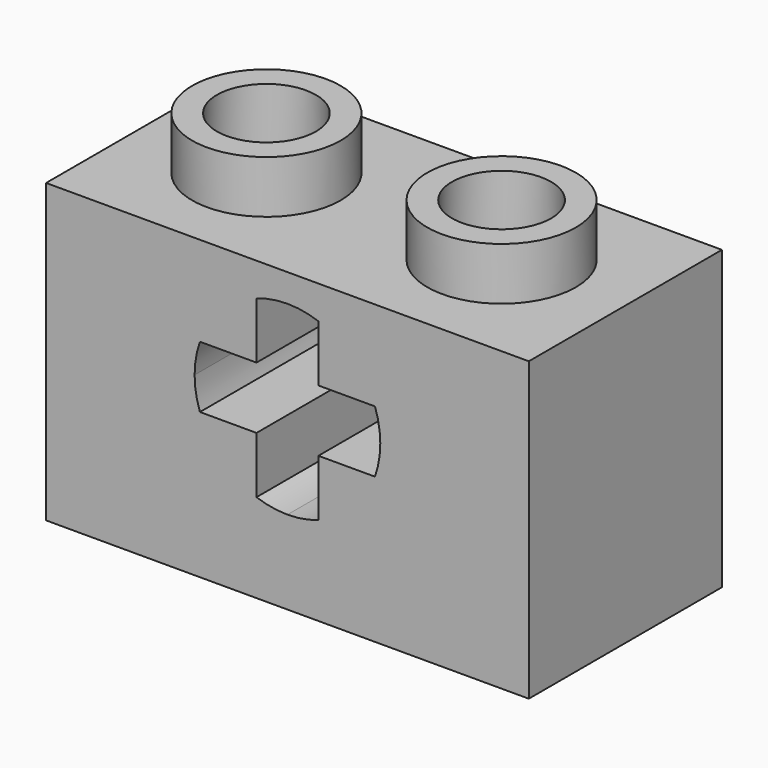
from build123d import *

# Parameters (mm, degrees)
F0_W     = 15.6
F0_H     = 9.6
F1_DEPTH = 7.8
F2_R     = 2.4
F2_R_2   = 1.6
F3_DEPTH = 1.7
F5_DEPTH = 2


# Not quite as in the source:
# - a feature names something its author has since deleted; it is built from what else it names


with BuildPart() as f1:
    # F0 (on Front) → F1 (new body)
    with BuildSketch(Plane.XZ):
        with Locations((7.5497636572, 4.7150965011)):
            Rectangle(F0_W, F0_H)
        with BuildLine():
            Line((10.5497636572, 6.6150965011), (10.5497636572, 5.6150965011))
            Line((10.5497636572, 5.6150965011), (10.5497636572, 4.6150965011))
            Line((10.5497636572, 4.6150965011), (10.3781907819, 4.6150965011))
            ThreePointArc((10.3781907819, 4.6150965011), (9.6710840007, 3.4937761575), (8.5497636572, 2.7866693764))
            Line((8.5497636572, 2.7866693764), (8.5497636572, 2.6150965011))
            Line((8.5497636572, 2.6150965011), (7.5497636572, 2.6150965011))
            Line((7.5497636572, 2.6150965011), (6.5497636572, 2.6150965011))
            Line((6.5497636572, 2.6150965011), (6.5497636572, 2.7866693764))
            ThreePointArc((6.5497636572, 2.7866693764), (5.4284433136, 3.4937761575), (4.7213365324, 4.6150965011))
            Line((4.7213365324, 4.6150965011), (4.5497636572, 4.6150965011))
            Line((4.5497636572, 4.6150965011), (4.5497636572, 5.6150965067))
            Line((4.5497636572, 5.6150965067), (4.5497636572, 6.6150965011))
            Line((4.5497636572, 6.6150965011), (4.7213365324, 6.6150965011))
            ThreePointArc((4.7213365324, 6.6150965011), (5.4284433136, 7.7364168447), (6.5497636572, 8.4435236258))
            Line((6.5497636572, 8.4435236258), (6.5497636572, 8.6150965011))
            Line((6.5497636572, 8.6150965011), (7.5497636572, 8.6150965011))
            Line((7.5497636572, 8.6150965011), (8.5497636572, 8.6150965011))
            Line((8.5497636572, 8.6150965011), (8.5497636572, 8.4435236258))
            ThreePointArc((8.5497636572, 8.4435236258), (9.6710840007, 7.7364168447), (10.3781907819, 6.6150965011))
            Line((10.3781907819, 6.6150965011), (10.5497636572, 6.6150965011))
        make_face(mode=Mode.SUBTRACT)
        with BuildLine():
            ThreePointArc((8.5497636572, 2.7866693764), (9.6710840007, 3.4937761575), (10.3781907819, 4.6150965011))
            Line((10.3781907819, 4.6150965011), (8.5497636572, 4.6150965011))
            Line((8.5497636572, 4.6150965011), (8.5497636572, 2.7866693764))
        make_face()
        with BuildLine():
            Line((8.5497636572, 6.6150965011), (10.3781907819, 6.6150965011))
            ThreePointArc((10.3781907819, 6.6150965011), (9.6710840007, 7.7364168447), (8.5497636572, 8.4435236258))
            Line((8.5497636572, 8.4435236258), (8.5497636572, 6.6150965011))
        make_face()
        with BuildLine():
            Line((4.7213365324, 6.6150965011), (6.5497636572, 6.6150965011))
            Line((6.5497636572, 6.6150965011), (6.5497636572, 8.4435236258))
            ThreePointArc((6.5497636572, 8.4435236258), (5.4284433136, 7.7364168447), (4.7213365324, 6.6150965011))
        make_face()
        with BuildLine():
            Line((6.5497636572, 2.7866693764), (6.5497636572, 4.6150965011))
            Line((6.5497636572, 4.6150965011), (4.7213365324, 4.6150965011))
            ThreePointArc((4.7213365324, 4.6150965011), (5.4284433136, 3.4937761575), (6.5497636572, 2.7866693764))
        make_face()
        with BuildLine():
            Line((10.5497636572, 4.6150965011), (10.5497636572, 5.6150965011))
            ThreePointArc((10.5497636572, 5.6150965011), (10.5065593361, 5.1077905649), (10.3781907819, 4.6150965011))
            Line((10.3781907819, 4.6150965011), (10.5497636572, 4.6150965011))
        make_face()
        with BuildLine():
            ThreePointArc((10.3781907819, 6.6150965011), (10.5065593361, 6.1224024373), (10.5497636572, 5.6150965011))
            Line((10.5497636572, 5.6150965011), (10.5497636572, 6.6150965011))
            Line((10.5497636572, 6.6150965011), (10.3781907819, 6.6150965011))
        make_face()
        with BuildLine():
            ThreePointArc((7.5497636572, 8.6150965011), (8.0570695933, 8.5718921801), (8.5497636572, 8.4435236258))
            Line((8.5497636572, 8.4435236258), (8.5497636572, 8.6150965011))
            Line((8.5497636572, 8.6150965011), (7.5497636572, 8.6150965011))
        make_face()
        with BuildLine():
            ThreePointArc((6.5497636572, 8.4435236258), (7.042457721, 8.5718921801), (7.5497636572, 8.6150965011))
            Line((7.5497636572, 8.6150965011), (6.5497636572, 8.6150965011))
            Line((6.5497636572, 8.6150965011), (6.5497636572, 8.4435236258))
        make_face()
        with BuildLine():
            ThreePointArc((4.5497636572, 5.6150965067), (4.5929679787, 6.12240244), (4.7213365324, 6.6150965011))
            Line((4.7213365324, 6.6150965011), (4.5497636572, 6.6150965011))
            Line((4.5497636572, 6.6150965011), (4.5497636572, 5.6150965067))
        make_face()
        with BuildLine():
            Line((4.5497636572, 4.6150965011), (4.7213365324, 4.6150965011))
            ThreePointArc((4.7213365324, 4.6150965011), (4.5929679777, 5.1077905677), (4.5497636572, 5.6150965067))
            Line((4.5497636572, 5.6150965067), (4.5497636572, 4.6150965011))
        make_face()
        with BuildLine():
            Line((6.5497636572, 2.6150965011), (7.5497636572, 2.6150965011))
            ThreePointArc((7.5497636572, 2.6150965011), (7.042457721, 2.6583008221), (6.5497636572, 2.7866693764))
            Line((6.5497636572, 2.7866693764), (6.5497636572, 2.6150965011))
        make_face()
        with BuildLine():
            Line((8.5497636572, 2.6150965011), (8.5497636572, 2.7866693764))
            ThreePointArc((8.5497636572, 2.7866693764), (8.0570695933, 2.6583008221), (7.5497636572, 2.6150965011))
            Line((7.5497636572, 2.6150965011), (8.5497636572, 2.6150965011))
        make_face()
    extrude(amount=F1_DEPTH)

    # F2 (on face) → F3 (join)
    with BuildSketch(Plane.XY.offset(9.5150965011)):
        with Locations((3.7497636572, -3.9)):
            Circle(F2_R)
        with Locations((3.7497636572, -3.9)):
            Circle(F2_R_2, mode=Mode.SUBTRACT)
        with Locations((11.3497636572, -3.9)):
            Circle(F2_R)
        with Locations((11.3497636572, -3.9)):
            Circle(F2_R_2, mode=Mode.SUBTRACT)
    extrude(amount=F3_DEPTH)

    # F4 (on face) → F5 (cut)
    with BuildSketch(Plane(origin=(0, 0, -0.0849034989), x_dir=(1, 0, 0), z_dir=(0, 0, -1))):
        Polygon((1.3497636572, 6.2), (1.3497636572, 3.9), (1.3497636572, 1.6), (7.5497636572, 1.6), (13.7497636572, 1.6), (13.7497636572, 3.9), (13.7497636572, 6.2), (7.5497636572, 6.2), align=None)
    extrude(amount=-F5_DEPTH, mode=Mode.SUBTRACT)


solid = f1.part
